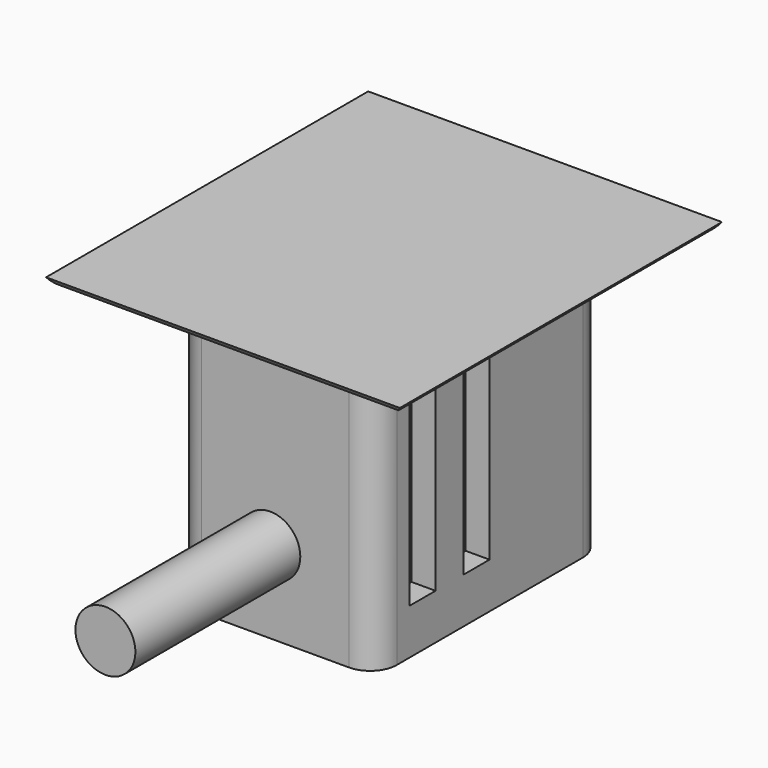
from build123d import *

# Parameters (mm, degrees)
F0_W         = 38.2822398096
F0_H         = 52.1388202906
F1_DEPTH     = 54.61
F2_R         = 5.728059517
F3_DEPTH     = 39.37
F4_W         = 6.2229996547
F4_H         = 34.6710011363
F5_DEPTH     = 4.572
F6_R         = 4.1653363511
F7_DEPTH     = 18.796
F8_W         = 67.563995719
F8_H         = 76.8984956667
F9_DEPTH     = 2.286
F10_T1_DEPTH = 64.8388202906
F10_T3_DEPTH = 88.7771779414
F10_T5_DEPTH = 98.1116778891


# Not quite as in the source:
# - a fillet or chamfer that OpenCascade refuses, or shapes differently, is made with other operations: its cross-section is extruded or revolved along the edge and cut away or added


with BuildPart() as f1:
    # F0 (on Front) → F1 (new body)
    with BuildSketch(Plane.XZ):
        with Locations((0.9477725253, -4.0886364877)):
            Rectangle(F0_W, F0_H)
    extrude(amount=-F1_DEPTH)

    # F2 (on Front) → F3 (join)
    with BuildSketch(Plane.XZ):
        with Locations((0, -14.5573755726)):
            Circle(F2_R)
    extrude(amount=F3_DEPTH)

    # F4 (on face) → F5 (cut)
    with BuildSketch(Plane.YZ.offset(20.0888924301)):
        with Locations((11.2236249261, -4.1116252542)):
            Rectangle(F4_W, F4_H)
        with Locations((24.1141221486, -4.1116252542)):
            Rectangle(F4_W, F4_H)
    extrude(amount=-F5_DEPTH, mode=Mode.SUBTRACT)

    # F6 (on face) → F7 (join)
    with BuildSketch(Plane(origin=(0, 54.61, 0), x_dir=(-1, 0, 0), z_dir=(0, 1, 0))):
        with Locations((0, 9.3980003148)):
            Circle(F6_R)
    extrude(amount=F7_DEPTH)

    # F8 (on face) → F9 (join)
    with BuildSketch(Plane.XY.offset(21.9807736576)):
        with Locations((0.1111254096, 27.0033725537)):
            Rectangle(F8_W, F8_H)
    extrude(amount=F9_DEPTH)

    # F10: fillet of radius 5.08 on 8 edges, made by hand

    # F10_s2 → F10_t1 (cut)
    with BuildSketch(Plane.XY.offset(-42.858046633)):
        with BuildLine():
            ThreePointArc((20.0888924301, 5.08), (18.6009948785, 1.4878975516), (15.0088924301, 0))
            Line((15.0088924301, 0), (20.0888924301, 0))
            Line((20.0888924301, 0), (20.0888924301, 5.08))
        make_face()
        with BuildLine():
            ThreePointArc((-18.1933473796, 5.08), (-16.705449828, 1.4878975516), (-13.1133473796, 0))
            Line((-13.1133473796, 0), (-18.1933473796, 0))
            Line((-18.1933473796, 0), (-18.1933473796, 5.08))
        make_face()
        with BuildLine():
            ThreePointArc((-13.1133473796, 54.61), (-16.705449828, 53.1221024484), (-18.1933473796, 49.53))
            Line((-18.1933473796, 49.53), (-18.1933473796, 54.61))
            Line((-18.1933473796, 54.61), (-13.1133473796, 54.61))
        make_face()
        with BuildLine():
            ThreePointArc((20.0888924301, 49.53), (18.6009948785, 53.1221024484), (15.0088924301, 54.61))
            Line((15.0088924301, 54.61), (20.0888924301, 54.61))
            Line((20.0888924301, 54.61), (20.0888924301, 49.53))
        make_face()
    extrude(amount=F10_T1_DEPTH, mode=Mode.SUBTRACT)

    # F10_s4 → F10_t3 (cut)
    with BuildSketch(Plane.YZ.offset(-44.2774635611)):
        with BuildLine():
            ThreePointArc((65.4526203871, 24.2667736576), (63.6196395196, 22.5886421747), (61.2099839426, 21.9807736576))
            Line((61.2099839426, 21.9807736576), (65.4526203871, 21.9807736576))
            Line((65.4526203871, 21.9807736576), (65.4526203871, 24.2667736576))
        make_face()
        with BuildLine():
            ThreePointArc((-11.4458752796, 24.2667736576), (-9.6128944122, 22.5886421747), (-7.2032388351, 21.9807736576))
            Line((-7.2032388351, 21.9807736576), (-11.4458752796, 21.9807736576))
            Line((-11.4458752796, 21.9807736576), (-11.4458752796, 24.2667736576))
        make_face()
    extrude(amount=F10_T3_DEPTH, mode=Mode.SUBTRACT)

    # F10_s6 → F10_t5 (cut)
    with BuildSketch(Plane.XZ.offset(-76.0592114983)):
        with BuildLine():
            ThreePointArc((29.6504868246, 21.9807736576), (32.0601424016, 22.5886421747), (33.8931232691, 24.2667736576))
            Line((33.8931232691, 24.2667736576), (33.8931232691, 21.9807736576))
            Line((33.8931232691, 21.9807736576), (29.6504868246, 21.9807736576))
        make_face()
        with BuildLine():
            ThreePointArc((-33.6708724499, 24.2667736576), (-31.8378915824, 22.5886421747), (-29.4282360054, 21.9807736576))
            Line((-29.4282360054, 21.9807736576), (-33.6708724499, 21.9807736576))
            Line((-33.6708724499, 21.9807736576), (-33.6708724499, 24.2667736576))
        make_face()
    extrude(amount=F10_T5_DEPTH, mode=Mode.SUBTRACT)


solid = f1.part
